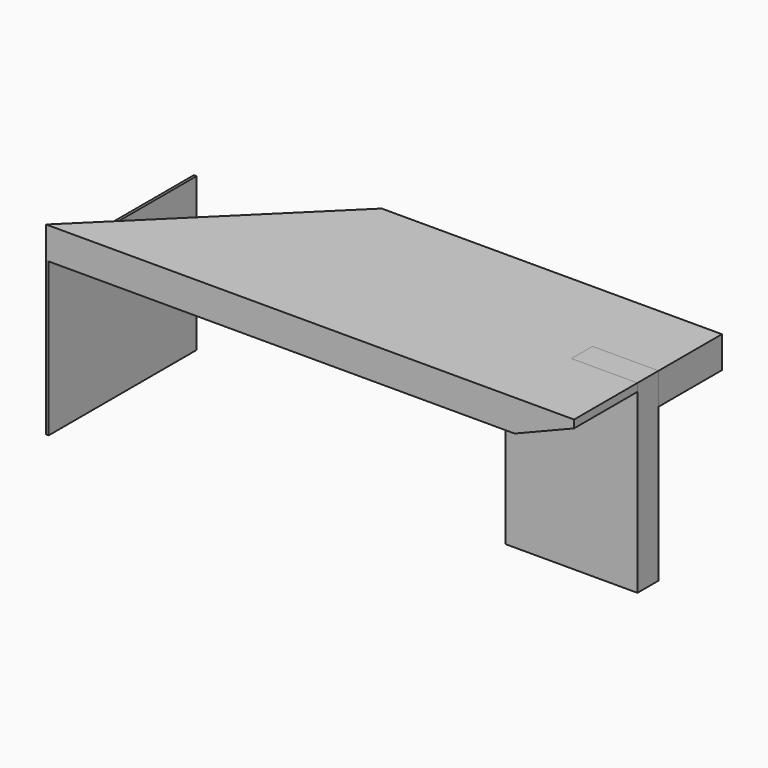
from build123d import *

# Parameters (mm, degrees)
F0_W      = 500
F0_H      = 700
F1_DEPTH  = 100
F2_W      = 250
F2_H      = 120
F3_DEPTH  = 231
F5_DEPTH  = 120
F6_W      = 10
F6_H      = 700
F7_DEPTH  = 580
F9_DEPTH  = 300
F11_DEPTH = 280


with BuildPart() as f1:
    # F0 (on Front) → F1 (new body)
    with BuildSketch(Plane.XZ):
        with Locations((17.2661517365, -13.1869101897)):
            Rectangle(F0_W, F0_H)
    extrude(amount=F1_DEPTH)

    # F2 (on face) → F3 (cut)
    with BuildSketch(Plane.XZ.offset(100)):
        with Locations((-107.7338482635, 276.8130898103)):
            Rectangle(F2_W, F2_H)
    extrude(amount=-F3_DEPTH, mode=Mode.SUBTRACT)


with BuildPart() as f5:
    # F4 (on face) → F5 (new body, through all)
    with BuildSketch(Plane.XY.offset(336.8130898103)):
        Polygon((17.2661517365, 0), (267.2661517365, 0), (267.2661517365, 300), (-1732.7338482635, 300), (-1732.7338482635, -400), (267.2661517365, -400), (267.2661517365, -100), (17.2661517365, -100), align=None)
    extrude(amount=-F5_DEPTH)

    # F8 (on face) → F9 (cut, through all)
    with BuildSketch(Plane.XZ.offset(400)):
        Polygon((267.2661517365, 307.2530031204), (42.1416759491, 216.8130898103), (267.2661517365, 216.8130898103), align=None)
    extrude(amount=-F9_DEPTH, mode=Mode.SUBTRACT)

    # F10 (on face) → F11 (cut)
    with BuildSketch(Plane.XY.offset(336.8130898103)):
        Polygon((-1732.7338482635, 300), (-1732.7338482635, -400), (-1021.2520360947, 300), align=None)
    extrude(amount=-F11_DEPTH, mode=Mode.SUBTRACT)


with BuildPart() as f7:
    # F6 (on face) → F7 (new body, through all)
    with BuildSketch(Plane(origin=(0, 0, 216.8130898103), x_dir=(1, 0, 0), z_dir=(0, 0, -1))):
        with Locations((-1727.7338482635, 50)):
            Rectangle(F6_W, F6_H)
    extrude(amount=F7_DEPTH)


solid = Compound([f1.part, f5.part, f7.part])
